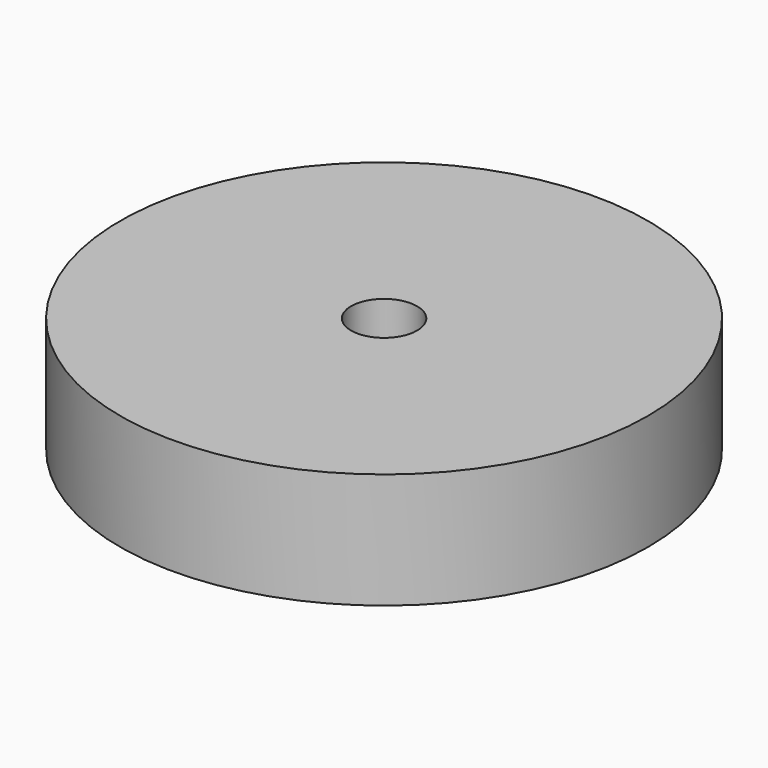
from build123d import *

# Parameters (mm, degrees)
F0_R     = 50.8
F1_DEPTH = 22.225
F2_R     = 6.35
F3_DEPTH = 22.225


# Not quite as in the source:
# - a length typed as a fraction of an inch, garbled in the dataset ("3 / 203.2 mm" for 3/8 in), is restored


with BuildPart() as f1:
    # F0 (on Top) → F1 (new body)
    with BuildSketch(Plane.XY):
        Circle(F0_R)
    extrude(amount=F1_DEPTH)

    # F2 (on face) → F3 (cut)
    with BuildSketch(Plane.XY.offset(22.225)):
        Circle(F2_R)
    extrude(amount=-F3_DEPTH, mode=Mode.SUBTRACT)


solid = f1.part
